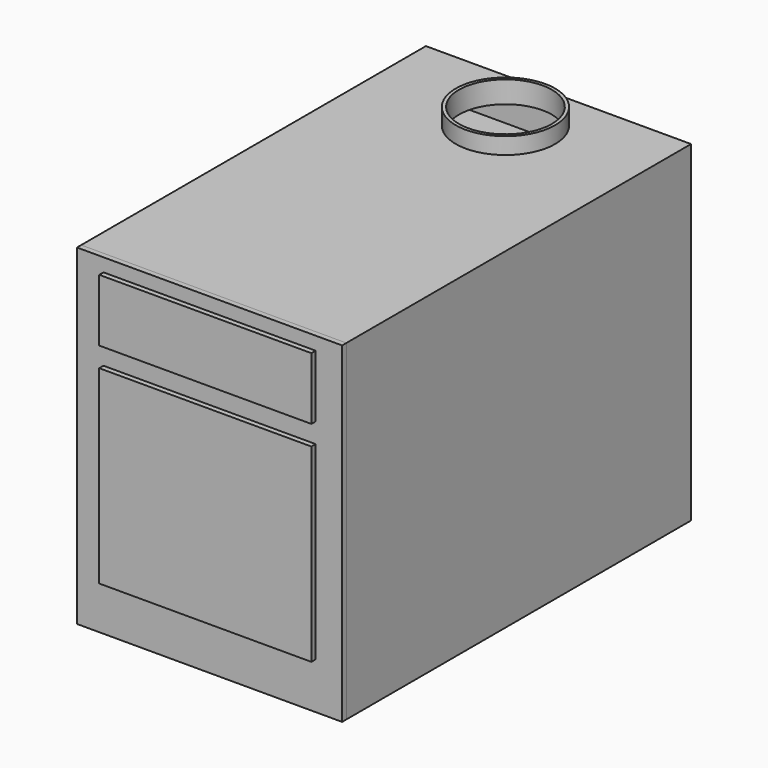
from build123d import *

# Parameters (mm, degrees)
F1_W      = 400
F1_H      = 650
F2_DEPTH  = 500
F3_T      = -8
F4_W      = 384
F4_H      = 8
F5_DEPTH  = 600
F6_W      = 384
F6_H      = 8
F7_DEPTH  = 600
F9_DEPTH  = 642
F10_R     = 75
F11_DEPTH = 25
F12_R     = 70
F13_DEPTH = 33
F14_W     = 400
F14_H     = 500
F14_W_2   = 300
F14_H_2   = 266
F14_H_3   = 74
F15_DEPTH = 8
F16_W     = 320
F16_H     = 94
F17_DEPTH = 8
F16_H_2   = 286


with BuildPart() as f2:
    # F1 (on Top) → F2 (new body)
    with BuildSketch(Plane.XY):
        with Locations((0, 325)):
            Rectangle(F1_W, F1_H)
    extrude(amount=F2_DEPTH)

    # F3
    f3_openings = [f2.faces().sort_by_distance(p)[0] for p in [
        (0, 0, 250),
    ]]
    offset(amount=F3_T, openings=f3_openings)

    # F10 (on face) → F11 (join)
    with BuildSketch(Plane.XY.offset(500)):
        with Locations((0, 550)):
            Circle(F10_R)
    extrude(amount=F11_DEPTH)

    # F12 (on face) → F13 (cut, through all)
    with BuildSketch(Plane.XY.offset(525)):
        with Locations((0, 550)):
            Circle(F12_R)
    extrude(amount=-F13_DEPTH, mode=Mode.SUBTRACT)


with BuildPart() as f5:
    # F4 (on face) → F5 (new body)
    with BuildSketch(Plane.XZ.offset(-642)):
        with Locations((0, 438)):
            Rectangle(F4_W, F4_H)
    extrude(amount=F5_DEPTH)


with BuildPart() as f7:
    # F6 (on face) → F7 (new body)
    with BuildSketch(Plane.XZ):
        with Locations((0, 380)):
            Rectangle(F6_W, F6_H)
    extrude(amount=-F7_DEPTH)


with BuildPart() as f9:
    # F8 (on face) → F9 (new body, through all)
    with BuildSketch(Plane.XZ.offset(-642)):
        Polygon((-167, 55), (-167, 58), (-192, 58), (-192, 33), (-189, 33), (-189, 55), align=None)
    extrude(amount=F9_DEPTH)


with BuildPart() as f9b:
    # F8 (on face) → F9, piece 2 (new body, through all)
    with BuildSketch(Plane.XZ.offset(-642)):
        Polygon((189, 33), (192, 33), (192, 58), (167, 58), (167, 55), (189, 55), align=None)
    extrude(amount=F9_DEPTH)


with BuildPart() as f15:
    # F14 (on face) → F15 (new body)
    with BuildSketch(Plane.XZ):
        with Locations((0, 250)):
            Rectangle(F14_W, F14_H)
        with Locations((0, 213)):
            Rectangle(F14_W_2, F14_H_2, mode=Mode.SUBTRACT)
        with Locations((0, 433)):
            Rectangle(F14_W_2, F14_H_3, mode=Mode.SUBTRACT)
    extrude(amount=F15_DEPTH)


with BuildPart() as f17:
    # F16 (on face) → F17 (new body)
    with BuildSketch(Plane.XZ.offset(8)):
        with Locations((0, 433)):
            Rectangle(F16_W, F16_H)
    extrude(amount=F17_DEPTH)


with BuildPart() as f17b:
    # F16 (on face) → F17, piece 2 (new body)
    with BuildSketch(Plane.XZ.offset(8)):
        with Locations((0, 213)):
            Rectangle(F16_W, F16_H_2)
    extrude(amount=F17_DEPTH)


solid = Compound([f2.part, f5.part, f7.part, f9.part, f9b.part, f15.part, f17.part, f17b.part])
